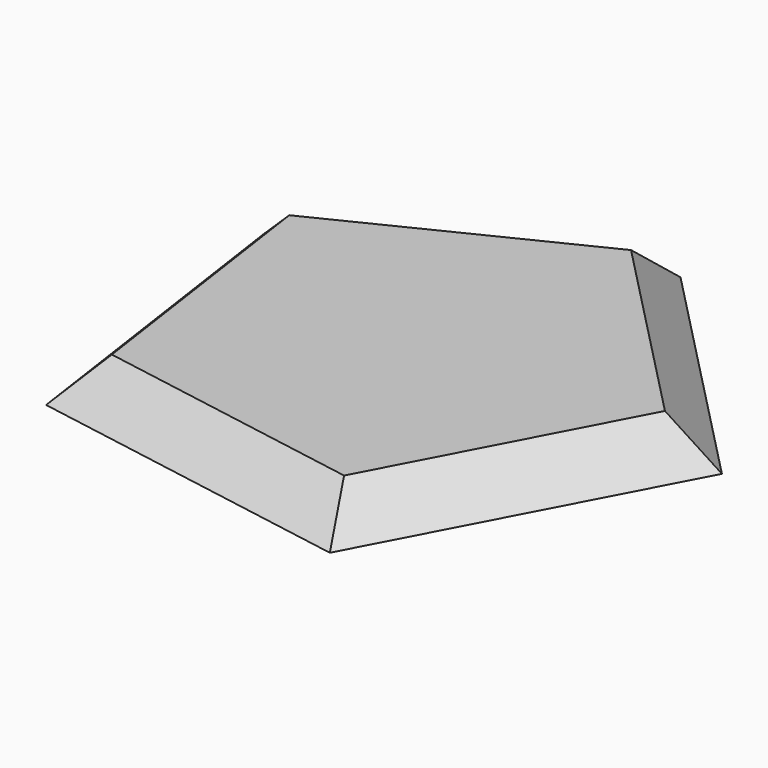
from build123d import *

# Parameters (mm, degrees)
F1_DEPTH = 6.35
F2_SIZE  = 6.34999


# Not quite as in the source:
# - a fillet or chamfer is up to 0.001 mm smaller than in the source, because OpenCascade refuses the exact size


with BuildPart() as f1:
    # F0 (on Top) → F1 (new body)
    with BuildSketch(Plane.XY):
        Polygon((7.3415196396, 42.584865104), (-38.2319591196, 20.141647113), (-30.9701698319, -30.1366425988), (19.0913415261, -38.7671165459), (42.7692677859, 6.1772469276), align=None)
    extrude(amount=F1_DEPTH)

    # F2 (size 6.35 in the source; OpenCascade refuses exactly that, so slightly less here)
    f2_edges = [f1.edges().sort_by_distance(p)[0] for p in [
        (30.930305, -16.294935, 6.35),
        (25.055394, 24.381056, 6.35),
        (-15.44522, 31.363256, 6.35),
        (-5.939414, -34.45188, 6.35),
        (-34.601064, -4.997498, 6.35),
    ]]
    chamfer(f2_edges, length=F2_SIZE)


solid = f1.part
